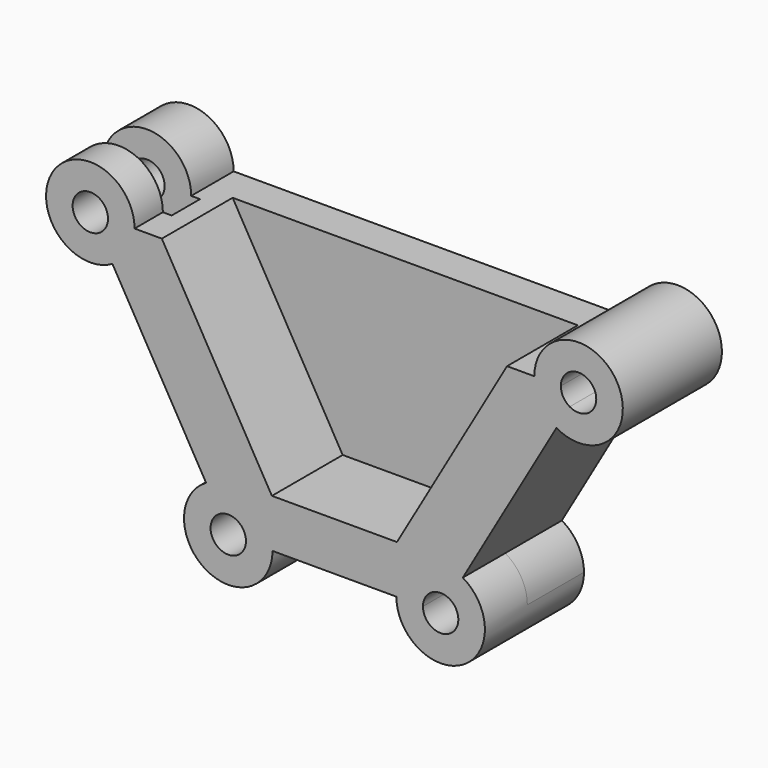
from build123d import *

# Parameters (mm, degrees)
F1_DEPTH  = 50.8
F3_DEPTH  = 76.2
F4_R      = 38.1
F1_FACE_R = 12.7
F5_DEPTH  = 12.7


with BuildPart() as f1:
    # F0 (on Front) → F1 (new body, symmetric)
    with BuildSketch(Plane.XZ):
        with BuildLine():
            ThreePointArc((-130.8751894546, 96.1189323328), (-190.1214960247, 111.9939323328), (-146.7501894546, 68.6226257627))
            Line((-146.7501894546, 68.6226257627), (-156.2751894546, 85.1204097048))
            ThreePointArc((-156.2751894546, 85.1204097048), (-173.6237120826, 102.4689323328), (-149.9251894546, 96.1189323328))
            Line((-149.9251894546, 96.1189323328), (-130.8751894546, 96.1189323328))
        make_face()
        with BuildLine():
            Line((-156.2751894546, 85.1204097048), (-146.7501894546, 68.6226257627))
            ThreePointArc((-146.7501894546, 68.6226257627), (-135.1288828844, 80.2439323328), (-130.8751894546, 96.1189323328))
            Line((-130.8751894546, 96.1189323328), (-149.9251894546, 96.1189323328))
            ThreePointArc((-149.9251894546, 96.1189323328), (-151.6266668265, 89.7689323328), (-156.2751894546, 85.1204097048))
        make_face()
        with BuildLine():
            Line((181.3982178505, 85.1204097048), (171.8732178505, 68.6226257627))
            ThreePointArc((171.8732178505, 68.6226257627), (203.6232178505, 68.6226257627), (219.4982178505, 96.1189323328))
            ThreePointArc((219.4982178505, 96.1189323328), (187.7482178505, 127.8689323328), (155.9982178505, 96.1189323328))
            Line((155.9982178505, 96.1189323328), (175.0482178505, 96.1189323328))
            ThreePointArc((175.0482178505, 96.1189323328), (187.7482178505, 108.8189323328), (200.4482178505, 96.1189323328))
            ThreePointArc((200.4482178505, 96.1189323328), (194.0982178505, 85.1204097048), (181.3982178505, 85.1204097048))
        make_face()
        with BuildLine():
            ThreePointArc((-79.513485802, -47.834761097), (-47.763485802, -47.834761097), (-31.888485802, -75.3310676672))
            Line((-31.888485802, -75.3310676672), (57.011514198, -75.3310676672))
            ThreePointArc((57.011514198, -75.3310676672), (72.886514198, -47.834761097), (104.636514198, -47.834761097))
            Line((104.636514198, -47.834761097), (171.8732178505, 68.6226257627))
            ThreePointArc((171.8732178505, 68.6226257627), (160.2519112804, 80.2439323328), (155.9982178505, 96.1189323328))
            Line((155.9982178505, 96.1189323328), (-130.8751894546, 96.1189323328))
            ThreePointArc((-130.8751894546, 96.1189323328), (-135.1288828844, 80.2439323328), (-146.7501894546, 68.6226257627))
            Line((-146.7501894546, 68.6226257627), (-79.513485802, -47.834761097))
        make_face()
        with BuildLine():
            Line((76.061514198, -75.3310676672), (57.011514198, -75.3310676672))
            ThreePointArc((57.011514198, -75.3310676672), (88.761514198, -107.0810676672), (120.511514198, -75.3310676672))
            ThreePointArc((120.511514198, -75.3310676672), (116.2578207681, -59.4560676672), (104.636514198, -47.834761097))
            Line((104.636514198, -47.834761097), (95.111514198, -64.3325450391))
            ThreePointArc((95.111514198, -64.3325450391), (99.760036826, -68.9810676672), (101.461514198, -75.3310676672))
            ThreePointArc((101.461514198, -75.3310676672), (88.761514198, -88.0310676672), (76.061514198, -75.3310676672))
        make_face()
        with BuildLine():
            ThreePointArc((104.636514198, -47.834761097), (72.886514198, -47.834761097), (57.011514198, -75.3310676672))
            Line((57.011514198, -75.3310676672), (76.061514198, -75.3310676672))
            ThreePointArc((76.061514198, -75.3310676672), (82.411514198, -64.3325450391), (95.111514198, -64.3325450391))
            Line((95.111514198, -64.3325450391), (104.636514198, -47.834761097))
        make_face()
        with BuildLine():
            Line((-31.888485802, -75.3310676672), (-50.938485802, -75.3310676672))
            ThreePointArc((-50.938485802, -75.3310676672), (-69.988485802, -86.3295902952), (-69.988485802, -64.3325450391))
            Line((-69.988485802, -64.3325450391), (-79.513485802, -47.834761097))
            ThreePointArc((-79.513485802, -47.834761097), (-79.513485802, -102.8273742373), (-31.888485802, -75.3310676672))
        make_face()
        with BuildLine():
            ThreePointArc((-69.988485802, -64.3325450391), (-57.288485802, -64.3325450391), (-50.938485802, -75.3310676672))
            Line((-50.938485802, -75.3310676672), (-31.888485802, -75.3310676672))
            ThreePointArc((-31.888485802, -75.3310676672), (-47.763485802, -47.834761097), (-79.513485802, -47.834761097))
            Line((-79.513485802, -47.834761097), (-69.988485802, -64.3325450391))
        make_face()
        with BuildLine():
            ThreePointArc((155.9982178505, 96.1189323328), (160.2519112804, 80.2439323328), (171.8732178505, 68.6226257627))
            Line((171.8732178505, 68.6226257627), (181.3982178505, 85.1204097048))
            ThreePointArc((181.3982178505, 85.1204097048), (176.7496952225, 89.7689323328), (175.0482178505, 96.1189323328))
            Line((175.0482178505, 96.1189323328), (155.9982178505, 96.1189323328))
        make_face()
    extrude(amount=F1_DEPTH, both=True)

    # F2 (on face) → F3 (cut)
    with BuildSketch(Plane.XZ.offset(50.8)):
        Polygon((136.4217789196, 96.1189323328), (-111.2987505236, 96.1189323328), (-32.3154252183, -40.6842000468), (57.4384536142, -40.6842000468), align=None)
    extrude(amount=-F3_DEPTH, mode=Mode.SUBTRACT)

    # F4 (on Front) + F1_face (on face) → F5 (cut, symmetric)
    with BuildSketch(Plane.XZ):
        with Locations((-162.6251894546, 96.1189323328)):
            Circle(F4_R)
    with BuildSketch(Plane(origin=(12.561514198, -50.8, 21.3503423812), x_dir=(1, 0, 0), z_dir=(0, -1, 0))):
        with BuildLine():
            Line((-123.8602647216, 74.7685899517), (-143.4367036526, 74.7685899517))
            ThreePointArc((-143.4367036526, 74.7685899517), (-202.6830102227, 90.6435899517), (-159.3117036526, 47.2722833815))
            Line((-159.3117036526, 47.2722833815), (-92.075, -69.1851034782))
            ThreePointArc((-92.075, -69.1851034782), (-92.075, -124.1777166185), (-44.45, -96.6814100483))
            Line((-44.45, -96.6814100483), (44.45, -96.6814100483))
            ThreePointArc((44.45, -96.6814100483), (92.075, -124.1777166185), (92.075, -69.1851034782))
            Line((92.075, -69.1851034782), (159.3117036526, 47.2722833815))
            ThreePointArc((159.3117036526, 47.2722833815), (202.6830102227, 90.6435899517), (143.4367036526, 74.7685899517))
            Line((143.4367036526, 74.7685899517), (123.8602647216, 74.7685899517))
            Line((123.8602647216, 74.7685899517), (44.8769394163, -62.0345424279))
            Line((44.8769394163, -62.0345424279), (-44.8769394163, -62.0345424279))
            Line((-44.8769394163, -62.0345424279), (-123.8602647216, 74.7685899517))
        make_face()
        with Locations((-76.2, -96.6814100483)):
            Circle(F1_FACE_R, mode=Mode.SUBTRACT)
        with Locations((76.2, -96.6814100483)):
            Circle(F1_FACE_R, mode=Mode.SUBTRACT)
        with Locations((-175.1867036526, 74.7685899517)):
            Circle(F1_FACE_R, mode=Mode.SUBTRACT)
        with Locations((175.1867036526, 74.7685899517)):
            Circle(F1_FACE_R, mode=Mode.SUBTRACT)
    extrude(amount=F5_DEPTH, both=True, mode=Mode.SUBTRACT)


solid = f1.part
